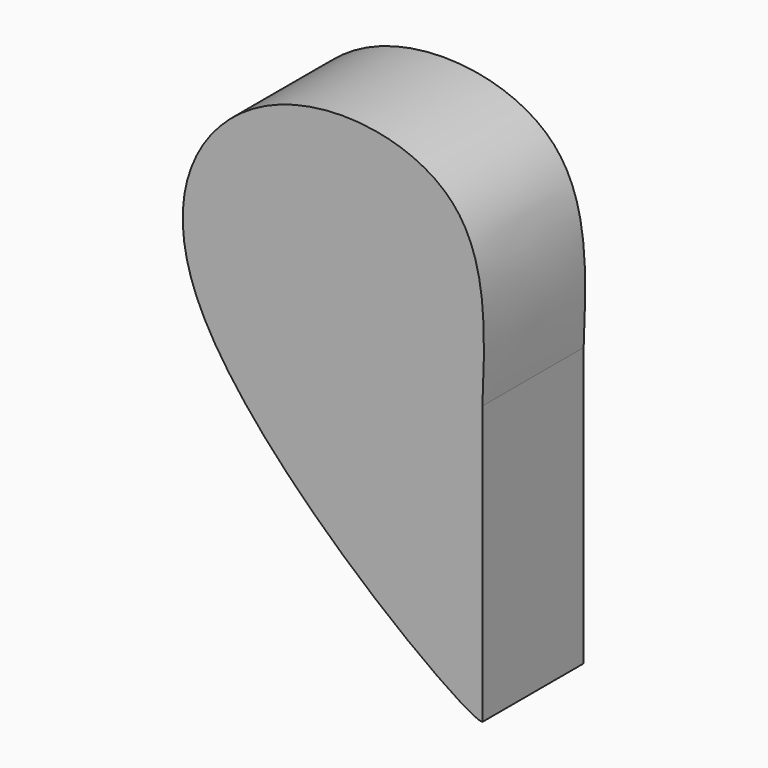
from build123d import *

# Parameters (mm, degrees)
F3_DEPTH = 25.4


# Not quite as in the source:
# - the dataset's text gives a spline's control points without its knots; the knots are read off the source's solid


with BuildPart() as f3:
    # F2 (on Front) → F3 (new body)
    with BuildSketch(Plane.XZ):
        with BuildLine():
            Line((0, -54.6992830932), (0, 0))
            add(Edge.make_bspline(
                [(0, 0), (0.5803927113, 13.3225663102), (1.7580073561, 40.3540036219), (-48.3152996398, 46.9838946285), (-76.9404589005, -2.5726478686), (-3.1471856567, -56.4537351882), (0, -55.8242015541)],
                knots=[0, 0, 0, 0, 0.2081992077, 0.4224354152, 0.6484719923, 0.9627025589, 0.9627025589, 0.9627025589, 0.9627025589], degree=3))
            Line((0, -55.8242015541), (0, -54.6992830932))
        make_face()
    extrude(amount=F3_DEPTH)


solid = f3.part
